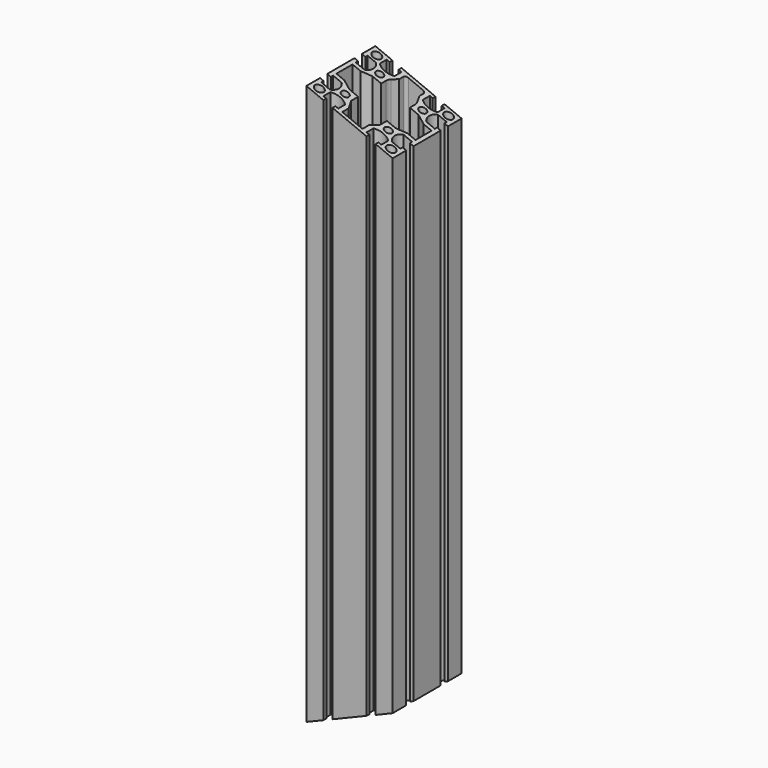
from build123d import *

# Parameters (mm, degrees)
F0_R          = 3
F0_R_2        = 2.5
F1_DEPTH      = 389.7
F2_R          = 2
F3_R          = 7
F5_DEPTH      = 30
F5_DEPTH_BACK = 30


# Not quite as in the source:
# - a feature names something its author has since deleted; it is built from what else it names


with BuildPart() as f1:
    # F0 (on Top) → F1 (new body)
    with BuildSketch(Plane.XY):
        with BuildLine():
            Line((18.15, -30), (30, -30))
            Line((30, -30), (30, -18.15))
            Line((30, -18.15), (27.5, -18.15))
            Line((27.5, -18.15), (27.5, -20.15))
            Line((27.5, -20.15), (21.5477069044, -20.15))
            ThreePointArc((21.5477069044, -20.15), (19.5, -15), (21.5477069044, -9.85))
            Line((21.5477069044, -9.85), (27.5, -9.85))
            Line((27.5, -9.85), (27.5, -11.85))
            Line((27.5, -11.85), (30, -11.85))
            Line((30, -11.85), (30, 11.85))
            Line((30, 11.85), (27.5, 11.85))
            Line((27.5, 11.85), (27.5, 9.85))
            Line((27.5, 9.85), (21.5477069044, 9.85))
            ThreePointArc((21.5477069044, 9.85), (19.5, 15), (21.5477069044, 20.15))
            Line((21.5477069044, 20.15), (27.5, 20.15))
            Line((27.5, 20.15), (27.5, 18.15))
            Line((27.5, 18.15), (30, 18.15))
            Line((30, 18.15), (30, 30))
            Line((30, 30), (18.15, 30))
            Line((18.15, 30), (18.15, 27.5))
            Line((18.15, 27.5), (20.15, 27.5))
            Line((20.15, 27.5), (20.15, 21.5477069044))
            ThreePointArc((20.15, 21.5477069044), (15, 19.5), (9.85, 21.5477069044))
            Line((9.85, 21.5477069044), (9.85, 27.5))
            Line((9.85, 27.5), (11.85, 27.5))
            Line((11.85, 27.5), (11.85, 30))
            Line((11.85, 30), (-11.85, 30))
            Line((-11.85, 30), (-11.85, 27.5))
            Line((-11.85, 27.5), (-9.85, 27.5))
            Line((-9.85, 27.5), (-9.85, 21.5477069044))
            ThreePointArc((-9.85, 21.5477069044), (-15, 19.5), (-20.15, 21.5477069044))
            Line((-20.15, 21.5477069044), (-20.15, 27.5))
            Line((-20.15, 27.5), (-18.15, 27.5))
            Line((-18.15, 27.5), (-18.15, 30))
            Line((-18.15, 30), (-30, 30))
            Line((-30, 30), (-30, 18.15))
            Line((-30, 18.15), (-27.5, 18.15))
            Line((-27.5, 18.15), (-27.5, 20.15))
            Line((-27.5, 20.15), (-21.5477069044, 20.15))
            ThreePointArc((-21.5477069044, 20.15), (-19.5, 15), (-21.5477069044, 9.85))
            Line((-21.5477069044, 9.85), (-27.5, 9.85))
            Line((-27.5, 9.85), (-27.5, 11.85))
            Line((-27.5, 11.85), (-30, 11.85))
            Line((-30, 11.85), (-30, -11.85))
            Line((-30, -11.85), (-27.5, -11.85))
            Line((-27.5, -11.85), (-27.5, -9.85))
            Line((-27.5, -9.85), (-21.5477069044, -9.85))
            ThreePointArc((-21.5477069044, -9.85), (-19.5, -15), (-21.5477069044, -20.15))
            Line((-21.5477069044, -20.15), (-27.5, -20.15))
            Line((-27.5, -20.15), (-27.5, -18.15))
            Line((-27.5, -18.15), (-30, -18.15))
            Line((-30, -18.15), (-30, -30))
            Line((-30, -30), (-18.15, -30))
            Line((-18.15, -30), (-18.15, -27.5))
            Line((-18.15, -27.5), (-20.15, -27.5))
            Line((-20.15, -27.5), (-20.15, -21.5477069044))
            ThreePointArc((-20.15, -21.5477069044), (-15, -19.5), (-9.85, -21.5477069044))
            Line((-9.85, -21.5477069044), (-9.85, -27.5))
            Line((-9.85, -27.5), (-11.85, -27.5))
            Line((-11.85, -27.5), (-11.85, -30))
            Line((-11.85, -30), (11.85, -30))
            Line((11.85, -30), (11.85, -27.5))
            Line((11.85, -27.5), (9.85, -27.5))
            Line((9.85, -27.5), (9.85, -21.5477069044))
            ThreePointArc((9.85, -21.5477069044), (15, -19.5), (20.15, -21.5477069044))
            Line((20.15, -21.5477069044), (20.15, -27.5))
            Line((20.15, -27.5), (18.15, -27.5))
            Line((18.15, -27.5), (18.15, -30))
        make_face()
        with Locations((-25, -25)):
            Circle(F0_R, mode=Mode.SUBTRACT)
        with Locations((-15, -15)):
            Circle(F0_R_2, mode=Mode.SUBTRACT)
        with Locations((25, -25)):
            Circle(F0_R, mode=Mode.SUBTRACT)
        with Locations((15, -15)):
            Circle(F0_R_2, mode=Mode.SUBTRACT)
        with Locations((-25, 25)):
            Circle(F0_R, mode=Mode.SUBTRACT)
        with Locations((-15, 15)):
            Circle(F0_R_2, mode=Mode.SUBTRACT)
        Polygon((-7, 22), (-7, 27.5), (0, 27.5), (7, 27.5), (7, 22), (10, 16), (10, 10), (16, 10), (22, 7), (27.5, 7), (27.5, 0), (27.5, -7), (22, -7), (16, -10), (10, -10), (10, -16), (7, -22), (7, -27.5), (0, -27.5), (-7, -27.5), (-7, -22), (-10, -16), (-10, -10), (-16, -10), (-22, -7), (-27.5, -7), (-27.5, 0), (-27.5, 7), (-22, 7), (-16, 10), (-10, 10), (-10, 16), align=None, mode=Mode.SUBTRACT)
        with Locations((15, 15)):
            Circle(F0_R_2, mode=Mode.SUBTRACT)
        with Locations((25, 25)):
            Circle(F0_R, mode=Mode.SUBTRACT)
    extrude(amount=F1_DEPTH)

    # F2
    f2_edges = [f1.edges().sort_by_distance(p)[0] for p in [
        (-7, 27.5, 194.85),
        (7, 27.5, 194.85),
    ]]
    fillet(f2_edges, radius=F2_R)

    # F3
    f3_edges = [f1.edges().sort_by_distance(p)[0] for p in [
        (-10, 16, 194.85),
        (10, 16, 194.85),
    ]]
    fillet(f3_edges, radius=F3_R)

    # F4 (on Front) → F5 (cut, two sides)
    with BuildSketch(Plane.XZ) as f5_sk:
        Polygon((262.6101504464, 391.20035759), (13.3822209239, 494.4339461204), (-30, 389.7), (219.2279295224, 286.4664114696), align=None)
        Polygon((237.6533260841, 110.8656376783), (-30, 0), (20.6125739706, -122.1895625065), (288.2659000547, -11.3239248282), align=None)
    extrude(amount=F5_DEPTH, mode=Mode.SUBTRACT)
    extrude(f5_sk.sketch, amount=-F5_DEPTH_BACK, mode=Mode.SUBTRACT)


solid = f1.part
